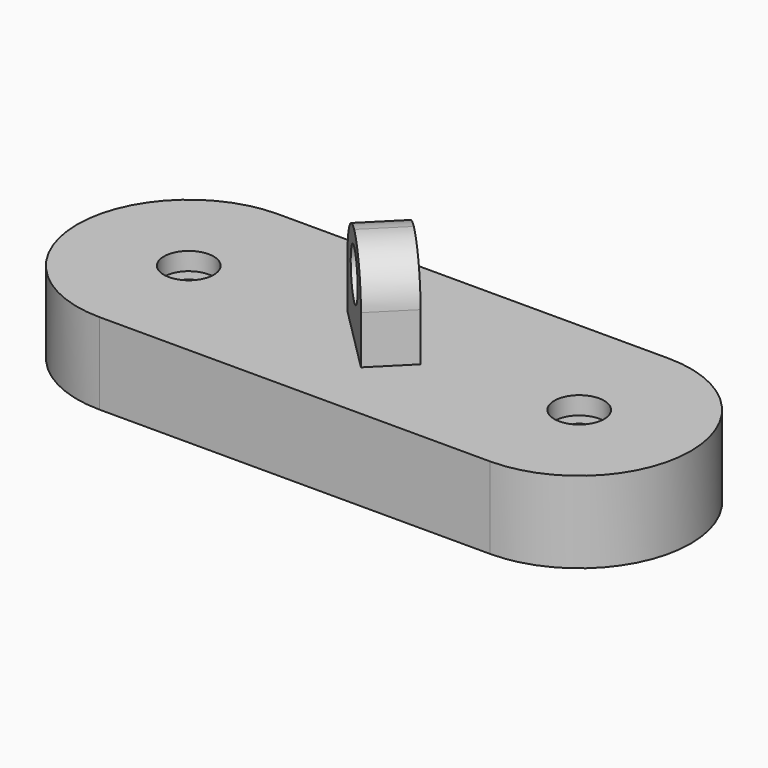
from build123d import *

# Parameters (mm, degrees)
F1_DEPTH     = 18.542
F2_R         = 5.6687062333
F3_DEPTH     = 4.064
F4_R         = 2.5242395044
F5_DEPTH     = 18.543
F8_W         = 21.7736046761
F8_H         = 40.5452698469
F9_DEPTH     = 5.334
F10_T1_DEPTH = 65.8569220358
F10_T3_DEPTH = 65.8569220358
F11_R        = 5.5506303957
F12_DEPTH    = 72.686920908


# Not quite as in the source:
# - a fillet or chamfer that OpenCascade refuses, or shapes differently, is made with other operations: its cross-section is extruded or revolved along the edge and cut away or added


with BuildPart() as f1:
    # F0 (on Top) → F1 (new body)
    with BuildSketch(Plane.XY):
        with BuildLine():
            Line((44.45, 25.4), (-44.45, 25.4))
            ThreePointArc((-44.45, 25.4), (-69.85, 0), (-44.45, -25.4))
            Line((-44.45, -25.4), (44.45, -25.4))
            ThreePointArc((44.45, -25.4), (69.85, 0), (44.45, 25.4))
        make_face()
    extrude(amount=F1_DEPTH)

    # F2 (on face) → F3 (cut)
    with BuildSketch(Plane.XY.offset(18.542)):
        with Locations((-44.45, 0)):
            Circle(F2_R)
        with Locations((44.45, 0)):
            Circle(F2_R)
    extrude(amount=-F3_DEPTH, mode=Mode.SUBTRACT)

    # F4 (on face) → F5 (cut, through all)
    with BuildSketch(Plane.XY.offset(18.542)):
        with Locations((-44.45, 0)):
            Circle(F4_R)
        with Locations((44.45, 0)):
            Circle(F4_R)
    extrude(amount=-F5_DEPTH, mode=Mode.SUBTRACT)

    # F8 (on line) → F9 (join, symmetric)
    with BuildSketch(Plane(origin=(0, 0, 0), x_dir=(-0.7071067812, 0.7071067812, 0), z_dir=(0.7071067812, 0.7071067812, 0))):
        with Locations((0, 20.2726349235)):
            Rectangle(F8_W, F8_H)
    extrude(amount=F9_DEPTH, both=True)

    # F10: fillet of radius 11.0377844072 on 2 edges, made by hand

    # F10_s2 → F10_t1 (cut)
    with BuildSketch(Plane(origin=(-23.2839380798, -23.2839380798, 0), x_dir=(0, 0, 1), z_dir=(0.7071067812, 0.7071067812, 0))):
        with BuildLine():
            ThreePointArc((29.5074854397, 10.8868023381), (37.3123776433, 7.6539101345), (40.5452698469, -0.1509820691))
            Line((40.5452698469, -0.1509820691), (40.5452698469, 10.8868023381))
            Line((40.5452698469, 10.8868023381), (29.5074854397, 10.8868023381))
        make_face()
    extrude(amount=F10_T1_DEPTH, mode=Mode.SUBTRACT)

    # F10_s4 → F10_t3 (cut)
    with BuildSketch(Plane(origin=(23.2839380798, 23.2839380798, 0), x_dir=(0, 0, 1), z_dir=(-0.7071067812, -0.7071067812, 0))):
        with BuildLine():
            ThreePointArc((29.5074854397, 10.8868023381), (37.3123776433, 7.6539101345), (40.5452698469, -0.1509820691))
            Line((40.5452698469, -0.1509820691), (40.5452698469, 10.8868023381))
            Line((40.5452698469, 10.8868023381), (29.5074854397, 10.8868023381))
        make_face()
    extrude(amount=F10_T3_DEPTH, mode=Mode.SUBTRACT)

    # F11 (on face) → F12 (cut, through all)
    with BuildSketch(Plane(origin=(3.7717075708, 3.7717075708, 0), x_dir=(-0.7071067812, 0.7071067812, 0), z_dir=(0.7071067812, 0.7071067812, 0))):
        with Locations((0, 31.5257720649)):
            Circle(F11_R)
    extrude(amount=-F12_DEPTH, mode=Mode.SUBTRACT)


solid = f1.part
